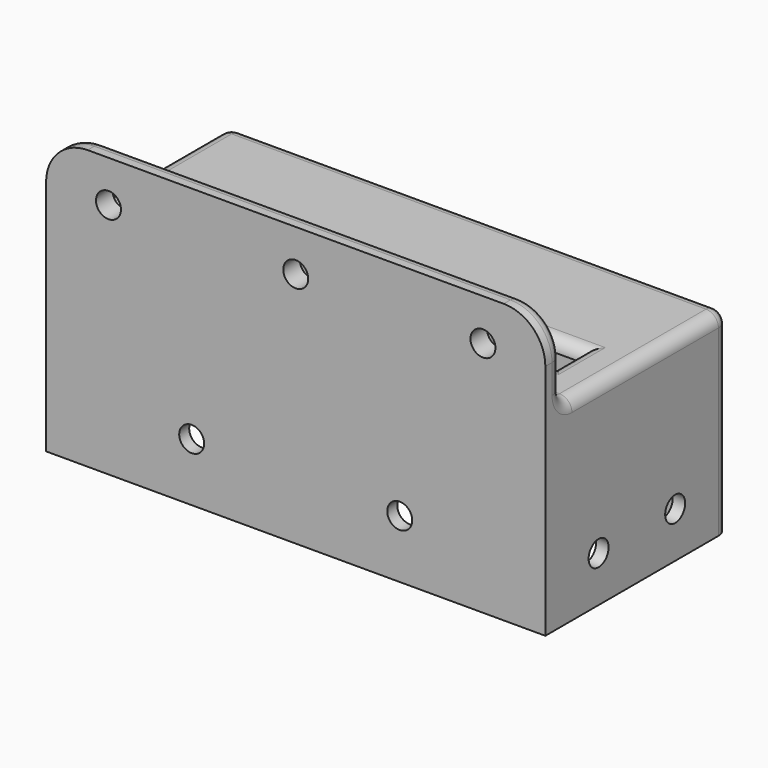
from build123d import *

# Parameters (mm, degrees)
F0_W      = 114
F0_H      = 49
F0_W_2    = 86
F0_H_2    = 8
F1_DEPTH  = 3
F0_W_3    = 120
F0_H_3    = 55
F2_DEPTH  = 47
F3_R      = 3
F4_DEPTH  = 130
F5_R      = 3
F6_DEPTH  = 10
F7_W      = 5
F7_H      = 20
F8_DEPTH  = 120
F9_R      = 3
F10_DEPTH = 25
F11_R     = 10
F12_R     = 2.99999


# Not quite as in the source:
# - a fillet or chamfer is up to 0.001 mm smaller than in the source, because OpenCascade refuses the exact size


with BuildPart() as f1:
    # F0 (on Top) → F1 (new body)
    with BuildSketch(Plane.XY):
        with Locations((60, 27.5)):
            Rectangle(F0_W, F0_H)
        with Locations((66, 21)):
            Rectangle(F0_W_2, F0_H_2, mode=Mode.SUBTRACT)
    extrude(amount=-F1_DEPTH)

    # F0 (on Top) → F2 (join)
    with BuildSketch(Plane.XY):
        with Locations((60, 27.5)):
            Rectangle(F0_W_3, F0_H_3)
        with Locations((60, 27.5)):
            Rectangle(F0_W, F0_H, mode=Mode.SUBTRACT)
    extrude(amount=-F2_DEPTH)

    # F3 (on Right) → F4 (cut)
    with BuildSketch(Plane.YZ):
        with Locations((39, -36)):
            Circle(F3_R)
        with Locations((16, -36)):
            Circle(F3_R)
    extrude(amount=F4_DEPTH, mode=Mode.SUBTRACT)

    # F5 (on Front) → F6 (cut)
    with BuildSketch(Plane.XZ):
        with Locations((35, -33)):
            Circle(F5_R)
        with Locations((85, -33)):
            Circle(F5_R)
    extrude(amount=-F6_DEPTH, mode=Mode.SUBTRACT)

    # F7 (on Right) → F8 (join)
    with BuildSketch(Plane.YZ):
        with Locations((2.5, 10)):
            Rectangle(F7_W, F7_H)
    extrude(amount=F8_DEPTH)

    # F9 (on Front) → F10 (cut)
    with BuildSketch(Plane.XZ):
        with Locations((15, 10)):
            Circle(F9_R)
        with Locations((60, 10)):
            Circle(F9_R)
        with Locations((105, 10)):
            Circle(F9_R)
    extrude(amount=-F10_DEPTH, mode=Mode.SUBTRACT)

    # F11
    f11_edges = [f1.edges().sort_by_distance(p)[0] for p in [
        (0, 2.5, 20),
        (120, 2.5, 20),
    ]]
    fillet(f11_edges, radius=F11_R)

    # F12 (radius 3 in the source; OpenCascade refuses exactly that, so slightly less here)
    f12_edges = [f1.edges().sort_by_distance(p)[0] for p in [
        (66, 17, 0),
        (60, 55, 0),
        (120, 30, 0),
        (60, 5, 0),
        (0, 30, 0),
        (109, 21, 0),
        (66, 25, 0),
        (23, 21, 0),
        (120, 55, -23.5),
        (0, 55, -23.5),
        (2.928932, 5, 17.071068),
        (60, 5, 20),
        (117.071068, 5, 17.071068),
    ]]
    fillet(f12_edges, radius=F12_R)


solid = f1.part
